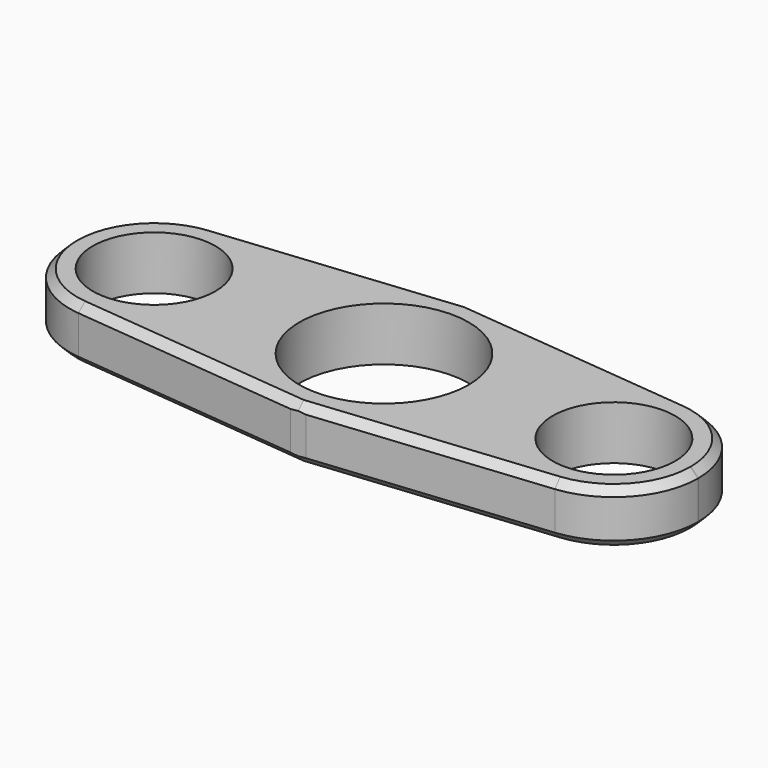
from build123d import *

# Parameters (mm, degrees)
F0_W         = 82
F0_H         = 28
F0_R         = 8
F0_R_2       = 11.05
F1_DEPTH     = 7
F2_SIZE2     = 4
F2_SIZE      = 40
F2_2_SIZE2   = 4
F2_2_SIZE    = 40
F3_R         = 11
F4_T1_DEPTH  = 43.1030542411
F4_T3_DEPTH  = 43.1030542411
F4_T5_DEPTH  = 43.1030542411
F4_T7_DEPTH  = 43.1030542411
F4_T9_DEPTH  = 0.0902736335
F4_T12_ANGLE = 84.2894068625
F4_T14_ANGLE = 84.2894068625
F4_T16_ANGLE = 84.2894068625
F4_T18_ANGLE = 84.2894068625
F4_T20_ANGLE = 84.2894068625
F4_T22_ANGLE = 84.2894068625
F4_T24_ANGLE = 84.2894068625
F4_T26_ANGLE = 84.2894068625


# Not quite as in the source:
# - a fillet or chamfer that OpenCascade refuses, or shapes differently, is made with other operations: its cross-section is extruded or revolved along the edge and cut away or added


with BuildPart() as f1:
    # F0 (on Top) → F1 (new body)
    with BuildSketch(Plane.XY):
        Rectangle(F0_W, F0_H)
        with Locations((-30, 0)):
            Circle(F0_R, mode=Mode.SUBTRACT)
        Circle(F0_R_2, mode=Mode.SUBTRACT)
        with Locations((30, 0)):
            Circle(F0_R, mode=Mode.SUBTRACT)
    extrude(amount=F1_DEPTH)

    # F2
    f2_edges = [f1.edges().sort_by_distance(p)[0] for p in [
        (-41, -14, 3.5),
        (41, -14, 3.5),
    ]]
    f2_side = f1.faces().sort_by_distance((0, -14, 3.5))[0]
    chamfer(f2_edges, length=F2_SIZE, length2=F2_SIZE2, reference=f2_side)

    # F2#2
    f2_2_edges = [f1.edges().sort_by_distance(p)[0] for p in [
        (41, 14, 3.5),
        (-41, 14, 3.5),
    ]]
    f2_2_side = f1.faces().sort_by_distance((0, 14, 3.5))[0]
    chamfer(f2_2_edges, length=F2_2_SIZE, length2=F2_2_SIZE2, reference=f2_2_side)

    # F3
    f3_edges = [f1.edges().sort_by_distance(p)[0] for p in [
        (-41, 10, 3.5),
        (-41, -10, 3.5),
        (41, 10, 3.5),
        (41, -10, 3.5),
    ]]
    fillet(f3_edges, radius=F3_R)

    # F4: chamfer of 1 on 20 edges, made by hand

    # F4_s2 → F4_t1 (cut)
    with BuildSketch(Plane(origin=(13.1906406762, -1.3190640676, 0), x_dir=(0, 0, 1), z_dir=(-0.9950371902, 0.099503719, 0))):
        Polygon((7, -13.030024382), (6, -14.030024382), (7, -14.030024382), align=None)
        Polygon((0, -13.030024382), (1, -14.030024382), (0, -14.030024382), align=None)
    extrude(amount=F4_T1_DEPTH, mode=Mode.SUBTRACT)

    # F4_s4 → F4_t3 (cut)
    with BuildSketch(Plane(origin=(-13.1906406762, -1.3190640676, 0), x_dir=(0, 0, 1), z_dir=(0.9950371902, 0.099503719, 0))):
        Polygon((7, 13.030024382), (6, 14.030024382), (7, 14.030024382), align=None)
        Polygon((0, 13.030024382), (1, 14.030024382), (0, 14.030024382), align=None)
    extrude(amount=F4_T3_DEPTH, mode=Mode.SUBTRACT)

    # F4_s6 → F4_t5 (cut)
    with BuildSketch(Plane(origin=(-13.1906406762, 1.3190640676, 0), x_dir=(0, 0, 1), z_dir=(0.9950371902, -0.099503719, 0))):
        Polygon((7, -13.030024382), (6, -14.030024382), (7, -14.030024382), align=None)
        Polygon((0, -13.030024382), (1, -14.030024382), (0, -14.030024382), align=None)
    extrude(amount=F4_T5_DEPTH, mode=Mode.SUBTRACT)

    # F4_s8 → F4_t7 (cut)
    with BuildSketch(Plane(origin=(13.1906406762, 1.3190640676, 0), x_dir=(0, 0, 1), z_dir=(-0.9950371902, -0.099503719, 0))):
        Polygon((7, 13.030024382), (6, 14.030024382), (7, 14.030024382), align=None)
        Polygon((0, 13.030024382), (1, 14.030024382), (0, 14.030024382), align=None)
    extrude(amount=F4_T7_DEPTH, mode=Mode.SUBTRACT)

    # F4_s10 → F4_t9 (cut)
    with BuildSketch(Plane.XZ.offset(-0.0451368168)):
        Polygon((41, 1), (40, 0), (41, 0), align=None)
        Polygon((41, 6), (40, 7), (41, 7), align=None)
        Polygon((-40, 0), (-41, 1), (-41, 0), align=None)
        Polygon((-40, 7), (-41, 6), (-41, 7), align=None)
    extrude(amount=F4_T9_DEPTH, mode=Mode.SUBTRACT)

    # F4_s11 → F4_t12 (revolve, cut)
    with BuildSketch(Plane.XZ.offset(0.0451368168)):
        Polygon((40, 0), (41, 1), (41, 0), align=None)
    revolve(axis=Axis((30, -0.0451368168, 0), (0, 0, -1)), revolution_arc=F4_T12_ANGLE, mode=Mode.SUBTRACT)

    # F4_s13 → F4_t14 (revolve, cut)
    with BuildSketch(Plane.XZ.offset(-0.0451368168)):
        Polygon((40, 0), (41, 1), (41, 0), align=None)
    revolve(axis=Axis((30, 0.0451368168, 0), (0, 0, 1)), revolution_arc=F4_T14_ANGLE, mode=Mode.SUBTRACT)

    # F4_s15 → F4_t16 (revolve, cut)
    with BuildSketch(Plane(origin=(-29.6985013053, 2.9698501305, 0), x_dir=(0, 0, 1), z_dir=(0.9950371902, -0.099503719, 0))):
        Polygon((0, 13.030024382), (1, 14.030024382), (0, 14.030024382), align=None)
    revolve(axis=Axis((-30, -0.0451368168, 0), (0, 0, -1)), revolution_arc=F4_T16_ANGLE, mode=Mode.SUBTRACT)

    # F4_s17 → F4_t18 (revolve, cut)
    with BuildSketch(Plane(origin=(-29.6985013053, -2.9698501305, 0), x_dir=(0, 0, 1), z_dir=(0.9950371902, 0.099503719, 0))):
        Polygon((0, -13.030024382), (1, -14.030024382), (0, -14.030024382), align=None)
    revolve(axis=Axis((-30, 0.0451368168, 0), (0, 0, 1)), revolution_arc=F4_T18_ANGLE, mode=Mode.SUBTRACT)

    # F4_s19 → F4_t20 (revolve, cut)
    with BuildSketch(Plane.XZ.offset(0.0451368168)):
        Polygon((41, 6), (40, 7), (41, 7), align=None)
    revolve(axis=Axis((30, -0.0451368168, 7), (0, 0, -1)), revolution_arc=F4_T20_ANGLE, mode=Mode.SUBTRACT)

    # F4_s21 → F4_t22 (revolve, cut)
    with BuildSketch(Plane.XZ.offset(-0.0451368168)):
        Polygon((41, 6), (40, 7), (41, 7), align=None)
    revolve(axis=Axis((30, 0.0451368168, 7), (0, 0, 1)), revolution_arc=F4_T22_ANGLE, mode=Mode.SUBTRACT)

    # F4_s23 → F4_t24 (revolve, cut)
    with BuildSketch(Plane(origin=(-29.6985013053, 2.9698501305, 0), x_dir=(0, 0, 1), z_dir=(0.9950371902, -0.099503719, 0))):
        Polygon((7, 13.030024382), (6, 14.030024382), (7, 14.030024382), align=None)
    revolve(axis=Axis((-30, -0.0451368168, 7), (0, 0, -1)), revolution_arc=F4_T24_ANGLE, mode=Mode.SUBTRACT)

    # F4_s25 → F4_t26 (revolve, cut)
    with BuildSketch(Plane(origin=(-29.6985013053, -2.9698501305, 0), x_dir=(0, 0, 1), z_dir=(0.9950371902, 0.099503719, 0))):
        Polygon((7, -13.030024382), (6, -14.030024382), (7, -14.030024382), align=None)
    revolve(axis=Axis((-30, 0.0451368168, 7), (0, 0, 1)), revolution_arc=F4_T26_ANGLE, mode=Mode.SUBTRACT)


solid = f1.part
